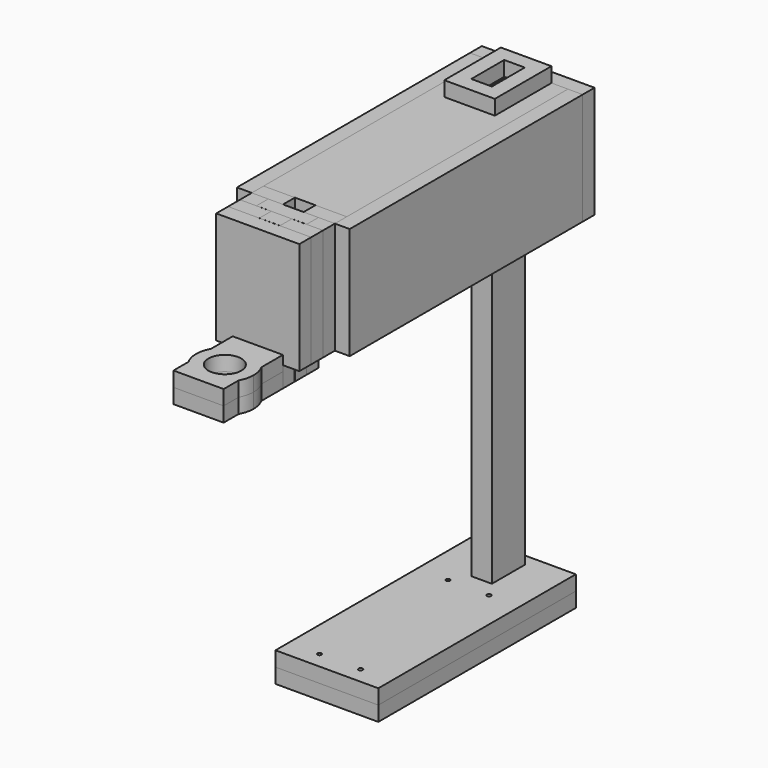
from build123d import *

# Parameters (mm, degrees)
F0_W      = 125
F0_H      = 300
F1_DEPTH  = 18
F2_DEPTH  = 18
F0_W_2    = 1
F0_H_2    = 1
F0_H_3    = 48
F3_DEPTH  = 550
F4_R      = 2.5
F5_DEPTH  = 36.001
F7_W      = 18
F7_H      = 50
F8_DEPTH  = 100
F7_H_2    = 18
F7_W_2    = 25
F9_DEPTH  = 100
F10_W     = 101
F10_H     = 336
F11_DEPTH = 18
F13_W     = 38
F13_H     = 50
F14_DEPTH = 18
F15_W     = 101
F15_H     = 118
F15_H_2   = 18
F16_DEPTH = 18
F17_DEPTH = 432.001
F18_W     = 25
F18_H     = 136
F19_DEPTH = 30
F18_W_2   = 20
F20_DEPTH = 18
F21_W     = 20
F21_H     = 136
F21_W_2   = 18
F22_DEPTH = 18
F21_W_3   = 38
F18_W_3   = 18
F23_DEPTH = 17.9
F24_DEPTH = 25
F25_W     = 61
F25_H     = 25
F26_DEPTH = 18
F27_W     = 25
F27_H     = 136
F28_DEPTH = 18
F30_DEPTH = 18
F31_W     = 61
F31_H     = 18
F32_DEPTH = 90
F33_R     = 20
F34_DEPTH = 18
F35_DEPTH = 24
F36_DEPTH = 18
F37_DEPTH = 18
F38_W     = 336
F38_H     = 136
F38_W_2   = 18
F39_DEPTH = 18
F40_W     = 354
F40_H     = 136
F41_DEPTH = 18
F42_W     = 137
F42_H     = 136
F43_DEPTH = 18
F44_W     = 61.4454383779
F44_H     = 86
F44_W_2   = 25
F44_H_2   = 50
F45_DEPTH = 18


with BuildPart() as f1:
    # F0 (on Top) → F1 (new body)
    with BuildSketch(Plane.XY):
        with Locations((2.1553742218, 30.5730341567)):
            Rectangle(F0_W, F0_H)
        Polygon((-10.3446257782, 164.5730341567), (-10.3446257782, 165.5730341567), (-9.3446257782, 165.5730341567), (14.6553742218, 165.5730341567), (14.6553742218, 115.5730341567), (-9.3446257782, 115.5730341567), (-10.3446257782, 115.5730341567), (-10.3446257782, 116.5730341567), align=None, mode=Mode.SUBTRACT)
    extrude(amount=F1_DEPTH)


with BuildPart() as f2:
    # F2 (new): a face of the model
    f2_faces = [f1.part.faces().sort_by_distance(p)[0] for p in [
        (2.1553742218, 26.7799307084, 18),
    ]]
    extrude(f2_faces, amount=F2_DEPTH)


with BuildPart() as f3:
    # F0 (on Top) → F3 (new body)
    with BuildSketch(Plane.XY):
        Polygon((14.6553742218, 165.5730341567), (-9.3446257782, 165.5730341567), (-9.3446257782, 164.5730341567), (13.6553742218, 164.5730341567), (13.6553742218, 116.5730341567), (-9.3446257782, 116.5730341567), (-9.3446257782, 115.5730341567), (14.6553742218, 115.5730341567), align=None)
        with Locations((-9.8446257782, 165.0730341567)):
            Rectangle(F0_W_2, F0_H_2)
        with Locations((-9.8446257782, 140.5730341567)):
            Rectangle(F0_W_2, F0_H_3)
        with Locations((-9.8446257782, 116.0730341567)):
            Rectangle(F0_W_2, F0_H_2)
    extrude(amount=F3_DEPTH)


with BuildPart() as f5_tool:
    # F4 (on face) → F5 (new body, through all)
    with BuildSketch(Plane.XY.offset(36)):
        with Locations((-22.8446257782, -99.4269658433)):
            Circle(F4_R)
        with Locations((27.1553742218, -99.4269658433)):
            Circle(F4_R)
        with Locations((27.1553742218, 95.5730341567)):
            Circle(F4_R)
        with Locations((-22.8446257782, 95.5730341567)):
            Circle(F4_R)
    extrude(amount=-F5_DEPTH)


with BuildPart() as f1_1:
    add(f1.part)

    # F5: cut by f5_tool
    add(f5_tool.part, mode=Mode.SUBTRACT)


with BuildPart() as f2_1:
    add(f2.part)

    # F5: cut by f5_tool
    add(f5_tool.part, mode=Mode.SUBTRACT)


with BuildPart() as f8:
    # F7 (on offset) → F8 (new body)
    with BuildSketch(Plane.XY.offset(432)):
        with Locations((-19.3446257782, 140.5730341567)):
            Rectangle(F7_W, F7_H)
    extrude(amount=F8_DEPTH)


with BuildPart() as f8b:
    # F7 (on offset) → F8, piece 2 (new body)
    with BuildSketch(Plane.XY.offset(432)):
        with Locations((23.6553742218, 140.5730341567)):
            Rectangle(F7_W, F7_H)
    extrude(amount=F8_DEPTH)


with BuildPart() as f9:
    # F7 (on offset) → F9 (new body)
    with BuildSketch(Plane.XY.offset(432)):
        with Locations((-19.3446257782, 106.5730341567)):
            Rectangle(F7_W, F7_H_2)
        with Locations((2.1553742218, 106.5730341567)):
            Rectangle(F7_W_2, F7_H_2)
        with Locations((23.6553742218, 106.5730341567)):
            Rectangle(F7_W, F7_H_2)
    extrude(amount=F9_DEPTH)


with BuildPart() as f9b:
    # F7 (on offset) → F9, piece 2 (new body)
    with BuildSketch(Plane.XY.offset(432)):
        with Locations((23.6553742218, 174.5730341567)):
            Rectangle(F7_W, F7_H_2)
        with Locations((2.1553742218, 174.5730341567)):
            Rectangle(F7_W_2, F7_H_2)
        with Locations((-19.3446257782, 174.5730341567)):
            Rectangle(F7_W, F7_H_2)
    extrude(amount=F9_DEPTH)


with BuildPart() as f11:
    # F10 (on offset) → F11 (new body)
    with BuildSketch(Plane.XY.offset(432)):
        with Locations((2.1553742218, 15.5730341567)):
            Rectangle(F10_W, F10_H)
    extrude(amount=-F11_DEPTH)

    # F7 (on offset) → F17 (cut, through all)
    with BuildSketch(Plane.XY.offset(432)):
        with Locations((2.1553742218, 140.5730341567)):
            Rectangle(F7_W_2, F7_H)
    extrude(amount=-F17_DEPTH, mode=Mode.SUBTRACT)


with BuildPart() as f14:
    # F13 (on offset) → F14 (new body)
    with BuildSketch(Plane.XY.offset(532)):
        Polygon((52.6553742218, 165.5730341567), (52.6553742218, 183.5730341567), (-48.3446257782, 183.5730341567), (-48.3446257782, 165.5730341567), (-10.3446257782, 165.5730341567), (14.6553742218, 165.5730341567), align=None)
        with Locations((33.6553742218, 140.5730341567)):
            Rectangle(F13_W, F13_H)
        with Locations((-29.3446257782, 140.5730341567)):
            Rectangle(F13_W, F13_H)
        Polygon((52.6553742218, -152.4269658433), (52.6553742218, 115.5730341567), (14.6553742218, 115.5730341567), (-10.3446257782, 115.5730341567), (-48.3446257782, 115.5730341567), (-48.3446257782, -152.4269658433), align=None)
    extrude(amount=F14_DEPTH)


with BuildPart() as f16:
    # F15 (on face) → F16 (new body)
    with BuildSketch(Plane.XZ.offset(152.4269658433)):
        with Locations((2.1553742218, 473)):
            Rectangle(F15_W, F15_H)
        with Locations((2.1553742218, 541)):
            Rectangle(F15_W, F15_H_2)
    extrude(amount=F16_DEPTH)

    # F18 (on face) → F19 (cut)
    with BuildSketch(Plane.XZ.offset(170.4269658433)):
        with Locations((2.1553742218, 482)):
            Rectangle(F18_W, F18_H)
    extrude(amount=-F19_DEPTH, mode=Mode.SUBTRACT)


with BuildPart() as f20:
    # F18 (on face) → F20 (new body)
    with BuildSketch(Plane.XZ.offset(170.4269658433)):
        with Locations((-38.3446257782, 482)):
            Rectangle(F18_W_2, F18_H)
    extrude(amount=F20_DEPTH)


with BuildPart() as f20b:
    # F18 (on face) → F20, piece 2 (new body)
    with BuildSketch(Plane.XZ.offset(170.4269658433)):
        with Locations((42.6553742218, 482)):
            Rectangle(F18_W_2, F18_H)
    extrude(amount=F20_DEPTH)


with BuildPart() as f22:
    # F21 (on face) → F22 (new body)
    with BuildSketch(Plane.XZ.offset(188.4269658433)):
        with Locations((-38.3446257782, 482)):
            Rectangle(F21_W, F21_H)
        with Locations((-19.3446257782, 482)):
            Rectangle(F21_W_2, F21_H)
    extrude(amount=F22_DEPTH)


with BuildPart() as f22b:
    # F21 (on face) → F22, piece 2 (new body)
    with BuildSketch(Plane.XZ.offset(188.4269658433)):
        with Locations((33.6553742218, 482)):
            Rectangle(F21_W_3, F21_H)
    extrude(amount=F22_DEPTH)


with BuildPart() as f23:
    # F18 (on face) → F23 (new body)
    with BuildSketch(Plane.XZ.offset(170.4269658433)):
        with Locations((-19.3446257782, 482)):
            Rectangle(F18_W_3, F18_H)
        with Locations((2.1553742218, 482)):
            Rectangle(F18_W, F18_H)
        with Locations((23.6553742218, 482)):
            Rectangle(F18_W_3, F18_H)
    extrude(amount=F23_DEPTH)

    # F24 (add): a face of the model
    f24_faces = [f23.faces().sort_by_distance(p)[0] for p in [
        (2.1553742218, -179.3769658433, 414),
    ]]
    extrude(f24_faces, amount=F24_DEPTH)


with BuildPart() as f26:
    # F25 (on face) → F26 (new body)
    with BuildSketch(Plane.XZ.offset(188.3269658433)):
        with Locations((2.1553742218, 401.5)):
            Rectangle(F25_W, F25_H)
    extrude(amount=F26_DEPTH)


with BuildPart() as f28:
    # F27 (on face) → F28 (new body)
    with BuildSketch(Plane.XZ.offset(188.3269658433)):
        with Locations((2.1553742218, 482)):
            Rectangle(F27_W, F27_H)
    extrude(amount=F28_DEPTH)


with BuildPart() as f30:
    # F29 (on face) → F30 (new body)
    with BuildSketch(Plane.XZ.offset(206.4269658433)):
        Polygon((52.6553742218, 550), (-10.3446257782, 550), (-10.3446257782, 414), (-28.3446257782, 414), (-28.3446257782, 389), (32.6553742218, 389), (32.6553742218, 414), (52.6553742218, 414), align=None)
        Polygon((-10.3446257782, 550), (-48.3446257782, 550), (-48.3446257782, 414), (-28.3446257782, 414), (-10.3446257782, 414), align=None)
    extrude(amount=F30_DEPTH)


with BuildPart() as f32:
    # F31 (on face) → F32 (new body)
    with BuildSketch(Plane.XZ.offset(224.4269658433)):
        with Locations((2.1553742218, 398)):
            Rectangle(F31_W, F31_H)
    extrude(amount=F32_DEPTH)

    # F33 (on face) → F34 (join)
    with BuildSketch(Plane.XY.offset(407)):
        with BuildLine():
            ThreePointArc((32.6553742218, -291.5952505567), (36.0116882563, -283.301085518), (37.1553742218, -274.4269658433))
            ThreePointArc((37.1553742218, -274.4269658433), (36.0116882563, -265.5528461687), (32.6553742218, -257.2586811299))
            Line((32.6553742218, -257.2586811299), (32.6553742218, -291.5952505567))
        make_face()
        with BuildLine():
            Line((32.6553742218, -291.5952505567), (32.6553742218, -257.2586811299))
            ThreePointArc((32.6553742218, -257.2586811299), (2.1553742218, -239.4269658433), (-28.3446257782, -257.2586811299))
            Line((-28.3446257782, -257.2586811299), (-28.3446257782, -291.5952505567))
            ThreePointArc((-28.3446257782, -291.5952505567), (2.1553742218, -309.4269658433), (32.6553742218, -291.5952505567))
        make_face()
        with Locations((2.1553742218, -274.4269658433)):
            Circle(F33_R, mode=Mode.SUBTRACT)
        with BuildLine():
            Line((-28.3446257782, -291.5952505567), (-28.3446257782, -257.2586811299))
            ThreePointArc((-28.3446257782, -257.2586811299), (-32.8446257782, -274.4269658433), (-28.3446257782, -291.5952505567))
        make_face()
    extrude(amount=-F34_DEPTH)

    # F33 (on face) → F35 (cut)
    with BuildSketch(Plane.XY.offset(407)):
        with Locations((2.1553742218, -274.4269658433)):
            Circle(F33_R)
    extrude(amount=-F35_DEPTH, mode=Mode.SUBTRACT)

    # F33 (on face) → F36 (join)
    with BuildSketch(Plane.XY.offset(407)):
        with BuildLine():
            Line((-28.3446257782, -291.5952505567), (-28.3446257782, -257.2586811299))
            ThreePointArc((-28.3446257782, -257.2586811299), (-32.8446257782, -274.4269658433), (-28.3446257782, -291.5952505567))
        make_face()
        with BuildLine():
            Line((32.6553742218, -291.5952505567), (32.6553742218, -257.2586811299))
            ThreePointArc((32.6553742218, -257.2586811299), (2.1553742218, -239.4269658433), (-28.3446257782, -257.2586811299))
            Line((-28.3446257782, -257.2586811299), (-28.3446257782, -291.5952505567))
            ThreePointArc((-28.3446257782, -291.5952505567), (2.1553742218, -309.4269658433), (32.6553742218, -291.5952505567))
        make_face()
        with Locations((2.1553742218, -274.4269658433)):
            Circle(F33_R, mode=Mode.SUBTRACT)
    extrude(amount=-F36_DEPTH)


with BuildPart() as f37:
    # F37 (new): a face of the model
    f37_faces = [f32.part.faces().sort_by_distance(p)[0] for p in [
        (2.1553742218, -225.5671412684, 407),
    ]]
    extrude(f37_faces, amount=F37_DEPTH)


with BuildPart() as f39:
    # F38 (on face) → F39 (new body)
    with BuildSketch(Plane(origin=(-48.3446257782, 0, 0), x_dir=(0, -1, 0), z_dir=(-1, 0, 0))):
        with Locations((-15.5730341567, 482)):
            Rectangle(F38_W, F38_H)
        with Locations((161.4269658433, 482)):
            Rectangle(F38_W_2, F38_H)
    extrude(amount=F39_DEPTH)


with BuildPart() as f41:
    # F40 (on face) → F41 (new body)
    with BuildSketch(Plane.YZ.offset(52.6553742218)):
        with Locations((6.5730341567, 482)):
            Rectangle(F40_W, F40_H)
    extrude(amount=F41_DEPTH)


with BuildPart() as f43:
    # F42 (on face) → F43 (new body)
    with BuildSketch(Plane(origin=(0, 183.5730341567, 0), x_dir=(-1, 0, 0), z_dir=(0, 1, 0))):
        with Locations((-2.1553742218, 482)):
            Rectangle(F42_W, F42_H)
    extrude(amount=F43_DEPTH)


with BuildPart() as f45:
    # F44 (on face) → F45 (new body)
    with BuildSketch(Plane.XY.offset(550)):
        with Locations((1.9326550329, 140.5730341567)):
            Rectangle(F44_W, F44_H)
        with Locations((2.1553742218, 140.5730341567)):
            Rectangle(F44_W_2, F44_H_2, mode=Mode.SUBTRACT)
    extrude(amount=F45_DEPTH)


with BuildPart() as f46_1:
    # F46: copy of F45
    add(f45.part.moved(Location((0, 0, -153.7))))


solid = Compound([f3.part, f1_1.part, f2_1.part, f8.part, f8b.part, f9.part, f9b.part, f11.part, f14.part, f16.part, f20.part, f20b.part, f22.part, f22b.part, f23.part, f26.part, f28.part, f30.part, f32.part, f37.part, f39.part, f41.part, f43.part, f45.part, f46_1.part])
